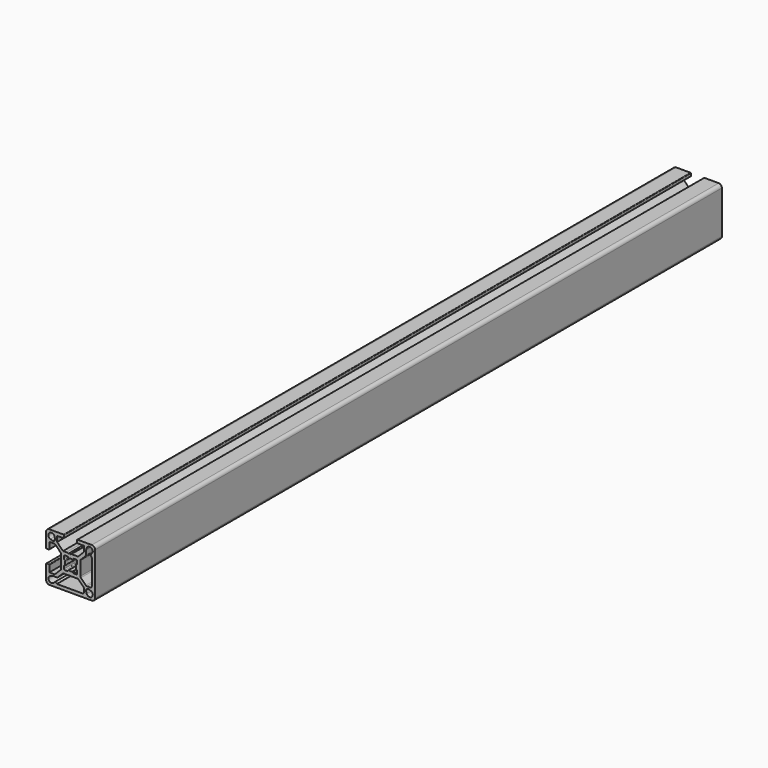
from build123d import *

# Parameters (mm, degrees)
F2_DEPTH = 240


# Not quite as in the source:
# - ends of sketch curves that miss each other by under 0.0002 mm in the source are joined


with BuildPart() as f2:
    # F1 (on Front) → F2 (new body, symmetric)
    with BuildSketch(Plane.XZ):
        with BuildLine():
            Line((-8.250056, 12.999986), (-4.300056, 12.999986))
            ThreePointArc((-4.300056, 12.999986), (-4.0879239656, 13.0878539656), (-4.000056, 13.299986))
            Line((-4.000056, 13.299986), (-4.000056, 14.699986))
            ThreePointArc((-4.000056, 14.699986), (-4.0879239656, 14.9121180344), (-4.300056, 14.999986))
            Line((-4.300056, 14.999986), (-13.000056, 14.999986))
            ThreePointArc((-13.000056, 14.999986), (-14.4142695624, 14.4141995624), (-15.000056, 12.999986))
            Line((-15.000056, 12.999986), (-15.000056, 4.299986))
            ThreePointArc((-15.000056, 4.299986), (-14.9121880344, 4.0878539656), (-14.700056, 3.999986))
            Line((-14.700056, 3.999986), (-13.300056, 3.999986))
            ThreePointArc((-13.300056, 3.999986), (-13.0879239656, 4.0878539656), (-13.000056, 4.299986))
            Line((-13.000056, 4.299986), (-13.000056, 8.249986))
            Line((-13.000056, 8.249986), (-9.66427, 8.249986))
            Line((-9.66427, 8.249986), (-6.000056, 4.585772))
            Line((-6.000056, 4.585772), (-6.000056, 0.653576))
            ThreePointArc((-6.000056, 0.653576), (-5.9830189324, 0.5241665494), (-5.9330687764, 0.4035761291))
            Line((-5.9330687764, 0.4035761291), (-5.700056, -1.4e-05))
            Line((-5.700056, -1.4e-05), (-5.933069, -0.403604))
            ThreePointArc((-5.933069, -0.403604), (-6.000056, -0.653604), (-5.9330687764, -0.9036038709))
            Line((-5.9330687764, -0.9036038709), (-5.751033, -1.2189))
            Line((-5.751033, -1.2189), (-6.000056, -2.500014))
            Line((-6.000056, -2.500014), (-6.000056, -4.5858))
            Line((-6.000056, -4.5858), (-9.66427, -8.250014))
            Line((-9.66427, -8.250014), (-13.000056, -8.250014))
            Line((-13.000056, -8.250014), (-13.000056, -4.300014))
            ThreePointArc((-13.000056, -4.300014), (-13.0879239656, -4.0878819656), (-13.300056, -4.000014))
            Line((-13.300056, -4.000014), (-14.700056, -4.000014))
            ThreePointArc((-14.700056, -4.000014), (-14.9121880344, -4.0878819656), (-15.000056, -4.300014))
            Line((-15.000056, -4.300014), (-15.000056, -13.000014))
            ThreePointArc((-15.000056, -13.000014), (-14.4142695624, -14.4142275624), (-13.000056, -15.000014))
            Line((-13.000056, -15.000014), (12.999944, -15.000014))
            ThreePointArc((12.999944, -15.000014), (14.4141575624, -14.4142275624), (14.999944, -13.000014))
            Line((14.999944, -13.000014), (14.999944, 12.999986))
            ThreePointArc((14.999944, 12.999986), (14.4141575624, 14.4141995624), (12.999944, 14.999986))
            Line((12.999944, 14.999986), (4.299944, 14.999986))
            ThreePointArc((4.299944, 14.999986), (4.0878119656, 14.9121180344), (3.999944, 14.699986))
            Line((3.999944, 14.699986), (3.999944, 13.299986))
            ThreePointArc((3.999944, 13.299986), (4.0878119656, 13.0878539656), (4.299944, 12.999986))
            Line((4.299944, 12.999986), (8.249944, 12.999986))
            Line((8.249944, 12.999986), (8.249944, 9.6642))
            Line((8.249944, 9.6642), (4.58573, 5.999986))
            Line((4.58573, 5.999986), (0.653534, 5.999986))
            ThreePointArc((0.653534, 5.999986), (0.5241245494, 5.9829489324), (0.4035341291, 5.9329987764))
            Line((0.4035341291, 5.9329987764), (-5.6e-05, 5.699986))
            Line((-5.6e-05, 5.699986), (-0.403646, 5.932999))
            ThreePointArc((-0.403646, 5.932999), (-0.653646, 5.999986), (-0.9036458709, 5.9329987764))
            Line((-0.9036458709, 5.9329987764), (-1.218942, 5.750963))
            Line((-1.218942, 5.750963), (-2.500056, 5.999986))
            Line((-2.500056, 5.999986), (-4.585842, 5.999986))
            Line((-4.585842, 5.999986), (-8.250056, 9.6642))
            Line((-8.250056, 9.6642), (-8.250056, 12.999986))
        make_face()
        with BuildLine():
            ThreePointArc((-8.189375, -13.000014), (-8.339375082, -12.9598215738), (-8.4491827159, -12.8500138359))
            ThreePointArc((-8.4491827159, -12.8500138359), (-9.2743948384, -12.3508472042), (-10.1375690315, -12.7810479782))
            ThreePointArc((-10.1375690315, -12.7810479782), (-13.2041723505, -12.8608903949), (-12.3498940253, -9.9145979306))
            Line((-12.3498940253, -9.9145979306), (-11.07346, -9.450014))
            Line((-11.07346, -9.450014), (-8.450056, -9.450014))
            ThreePointArc((-8.450056, -9.450014), (-8.0673725676, -9.3738935325), (-7.7429492188, -9.1571207812))
            Line((-7.7429492188, -9.1571207812), (-4.878736, -6.292907))
            ThreePointArc((-4.878736, -6.292907), (-4.5543124324, -6.0761344675), (-4.171629, -6.000014))
            Line((-4.171629, -6.000014), (4.171517, -6.000014))
            ThreePointArc((4.171517, -6.000014), (4.5542004324, -6.0761344675), (4.8786237812, -6.2929072188))
            Line((4.8786237812, -6.2929072188), (7.957051, -9.371334))
            ThreePointArc((7.957051, -9.371334), (8.1738235325, -9.6957575676), (8.249944, -10.078441))
            Line((8.249944, -10.078441), (8.249944, -12.000014))
            ThreePointArc((8.249944, -12.000014), (7.9570507812, -12.7071207812), (7.249944, -13.000014))
            Line((7.249944, -13.000014), (-8.189375, -13.000014))
        make_face(mode=Mode.SUBTRACT)
        with BuildLine():
            ThreePointArc((9.5477956661, -11.3422641215), (9.8734155063, -9.8734855063), (11.3421941215, -9.5478656661))
            Line((11.3421941215, -9.5478656661), (12.349782, -9.914598))
            ThreePointArc((12.349782, -9.914598), (13.0434468843, -13.0435168843), (9.9145279306, -12.3498520253))
            Line((9.9145279306, -12.3498520253), (9.5477956661, -11.3422641215))
        make_face(mode=Mode.SUBTRACT)
        with BuildLine():
            ThreePointArc((-9.5479076661, 11.3422361215), (-9.8735275063, 9.8734575063), (-11.3423061215, 9.5478376661))
            Line((-11.3423061215, 9.5478376661), (-12.349894, 9.91457))
            ThreePointArc((-12.349894, 9.91457), (-13.0435588843, 13.0434888843), (-9.9146399306, 12.3498240253))
            Line((-9.9146399306, 12.3498240253), (-9.5479076661, 11.3422361215))
        make_face(mode=Mode.SUBTRACT)
        with BuildLine():
            ThreePointArc((3.2531309855, 0.9883049956), (3.399944, -1.4e-05), (3.2531309855, -0.9883329956))
            ThreePointArc((3.2531309855, -0.9883329956), (3.2974111593, -1.3177976431), (3.5754529349, -1.5000144258))
            ThreePointArc((3.5754529349, -1.5000144258), (3.8792555231, -1.6685151025), (3.999944, -1.99428))
            Line((3.999944, -1.99428), (3.999944, -3.500014))
            ThreePointArc((3.999944, -3.500014), (3.8534973906, -3.8535673906), (3.499944, -4.000014))
            Line((3.499944, -4.000014), (1.99421, -4.000014))
            ThreePointArc((1.99421, -4.000014), (1.6684451025, -3.8793255231), (1.4999444822, -3.5755229263))
            ThreePointArc((1.4999444822, -3.5755229263), (1.3177276431, -3.2974811593), (0.9882590481, -3.2532021585))
            ThreePointArc((0.9882590481, -3.2532021585), (-5.6e-05, -3.400014), (-0.9883749956, -3.2532009855))
            ThreePointArc((-0.9883749956, -3.2532009855), (-1.3178396431, -3.2974811593), (-1.5000564258, -3.5755229349))
            ThreePointArc((-1.5000564258, -3.5755229349), (-1.6685571025, -3.8793255231), (-1.994322, -4.000014))
            Line((-1.994322, -4.000014), (-3.500056, -4.000014))
            ThreePointArc((-3.500056, -4.000014), (-3.8536093906, -3.8535673906), (-4.000056, -3.500014))
            Line((-4.000056, -3.500014), (-4.000056, -1.99428))
            ThreePointArc((-4.000056, -1.99428), (-3.8793675231, -1.6685151025), (-3.5755649263, -1.5000144822))
            ThreePointArc((-3.5755649263, -1.5000144822), (-3.2975231593, -1.3177976431), (-3.2532441585, -0.9883290481))
            ThreePointArc((-3.2532441585, -0.9883290481), (-3.400056, -1.4e-05), (-3.2532429855, 0.9883049956))
            ThreePointArc((-3.2532429855, 0.9883049956), (-3.2975231593, 1.3177696431), (-3.5755649349, 1.4999864258))
            ThreePointArc((-3.5755649349, 1.4999864258), (-3.8793675231, 1.6684871025), (-4.000056, 1.994252))
            Line((-4.000056, 1.994252), (-4.000056, 3.499986))
            ThreePointArc((-4.000056, 3.499986), (-3.8536093906, 3.8535393906), (-3.500056, 3.999986))
            Line((-3.500056, 3.999986), (-1.994322, 3.999986))
            ThreePointArc((-1.994322, 3.999986), (-1.6685571025, 3.8792975231), (-1.5000564822, 3.5754949263))
            ThreePointArc((-1.5000564822, 3.5754949263), (-1.3178396431, 3.2974531593), (-0.9883710481, 3.2531741585))
            ThreePointArc((-0.9883710481, 3.2531741585), (-5.6e-05, 3.399986), (0.9882629956, 3.2531729855))
            ThreePointArc((0.9882629956, 3.2531729855), (1.3177276431, 3.2974531593), (1.4999444258, 3.5754949349))
            ThreePointArc((1.4999444258, 3.5754949349), (1.6684451025, 3.8792975231), (1.99421, 3.999986))
            Line((1.99421, 3.999986), (3.499944, 3.999986))
            ThreePointArc((3.499944, 3.999986), (3.8534973906, 3.8535393906), (3.999944, 3.499986))
            Line((3.999944, 3.499986), (3.999944, 1.994252))
            ThreePointArc((3.999944, 1.994252), (3.8792555231, 1.6684871025), (3.5754529263, 1.4999864822))
            ThreePointArc((3.5754529263, 1.4999864822), (3.2974111593, 1.3177696431), (3.2531309855, 0.9883049956))
        make_face(mode=Mode.SUBTRACT)
        with BuildLine():
            ThreePointArc((6.2928372188, -4.8786937812), (6.0760644675, -4.5542704324), (5.999944, -4.171587))
            Line((5.999944, -4.171587), (5.999944, 4.171559))
            ThreePointArc((5.999944, 4.171559), (6.0760644675, 4.5542424324), (6.2928372188, 4.8786657812))
            Line((6.2928372188, 4.8786657812), (9.157051, 7.742879))
            ThreePointArc((9.157051, 7.742879), (9.3738235325, 8.0673025676), (9.449944, 8.449986))
            Line((9.449944, 8.449986), (9.449944, 11.07339))
            Line((9.449944, 11.07339), (9.914528, 12.349824))
            ThreePointArc((9.914528, 12.349824), (12.8608203949, 13.2041023505), (12.7809779799, 10.1374990291))
            ThreePointArc((12.7809779799, 10.1374990291), (12.3507772042, 9.2743248384), (12.8499438252, 8.4491126972))
            ThreePointArc((12.8499438252, 8.4491126972), (12.9597515738, 8.339305082), (12.999944, 8.189305))
            Line((12.999944, 8.189305), (12.999944, -7.250014))
            ThreePointArc((12.999944, -7.250014), (12.7070507812, -7.9571207812), (11.999944, -8.250014))
            Line((11.999944, -8.250014), (10.078371, -8.250014))
            ThreePointArc((10.078371, -8.250014), (9.6956875676, -8.1738935325), (9.3712642188, -7.9571207812))
            Line((9.3712642188, -7.9571207812), (6.2928372188, -4.8786937812))
        make_face(mode=Mode.SUBTRACT)
    extrude(amount=F2_DEPTH, both=True)


solid = f2.part
